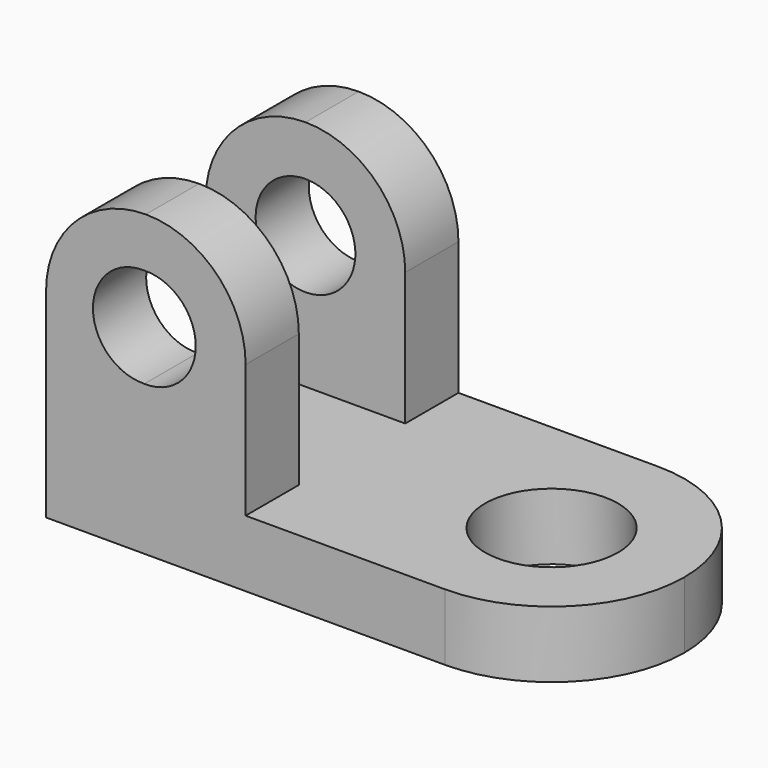
from build123d import *

# Parameters (mm, degrees)
F0_W      = 101.6
F0_H      = 50.8
F1_DEPTH  = 12.7
F3_R      = 25.39999
F2_R      = 12.7
F4_DEPTH  = 12.701
F5_W      = 38.1
F5_H      = 12.7
F6_DEPTH  = 44.45
F7_R      = 19.04999
F8_R      = 9.525
F9_DEPTH  = 50.801
F10_W     = 38.1
F10_H     = 12.7
F11_DEPTH = 44.45
F12_R     = 19.04999
F13_R     = 9.525
F14_DEPTH = 50.801


# Not quite as in the source:
# - a fillet or chamfer is up to 0.001 mm smaller than in the source, because OpenCascade refuses the exact size


with BuildPart() as f1:
    # F0 (on Top) → F1 (new body)
    with BuildSketch(Plane.XY):
        with Locations((11.9383526917, -1.5475824475)):
            Rectangle(F0_W, F0_H)
    extrude(amount=F1_DEPTH)

    # F3 (radius 25.4 in the source; OpenCascade refuses exactly that, so slightly less here)
    f3_edges = [f1.edges().sort_by_distance(p)[0] for p in [
        (62.738353, -26.947582, 6.35),
        (62.738353, 23.852418, 6.35),
    ]]
    fillet(f3_edges, radius=F3_R)

    # F2 (on face) → F4 (cut, through all)
    with BuildSketch(Plane.XY.offset(12.7)):
        with Locations((37.3383526917, -1.5475824475)):
            Circle(F2_R)
    extrude(amount=-F4_DEPTH, mode=Mode.SUBTRACT)

    # F5 (on face) → F6 (join)
    with BuildSketch(Plane.XY.offset(12.7)):
        with Locations((-19.8116473083, -20.5975824475)):
            Rectangle(F5_W, F5_H)
    extrude(amount=F6_DEPTH)

    # F7 (radius 19.05 in the source; OpenCascade refuses exactly that, so slightly less here)
    f7_edges = [f1.edges().sort_by_distance(p)[0] for p in [
        (-38.861647, -20.597582, 57.15),
        (-0.761647, -20.597582, 57.15),
    ]]
    fillet(f7_edges, radius=F7_R)

    # F8 (on face) → F9 (cut, through all)
    with BuildSketch(Plane.XZ.offset(26.9475824475)):
        with Locations((-20.3908979893, 38.1)):
            Circle(F8_R)
    extrude(amount=-F9_DEPTH, mode=Mode.SUBTRACT)

    # F10 (on face) → F11 (join)
    with BuildSketch(Plane.XY.offset(12.7)):
        with Locations((-19.8116473083, 17.5024175525)):
            Rectangle(F10_W, F10_H)
    extrude(amount=F11_DEPTH)

    # F12 (radius 19.05 in the source; OpenCascade refuses exactly that, so slightly less here)
    f12_edges = [f1.edges().sort_by_distance(p)[0] for p in [
        (-0.761647, 17.502418, 57.15),
        (-38.861647, 17.502418, 57.15),
    ]]
    fillet(f12_edges, radius=F12_R)

    # F13 (on face) → F14 (cut, through all)
    with BuildSketch(Plane(origin=(0, 23.8524175525, 0), x_dir=(-1, 0, 0), z_dir=(0, 1, 0))):
        with Locations((19.8116473083, 38.1)):
            Circle(F13_R)
    extrude(amount=-F14_DEPTH, mode=Mode.SUBTRACT)


solid = f1.part
